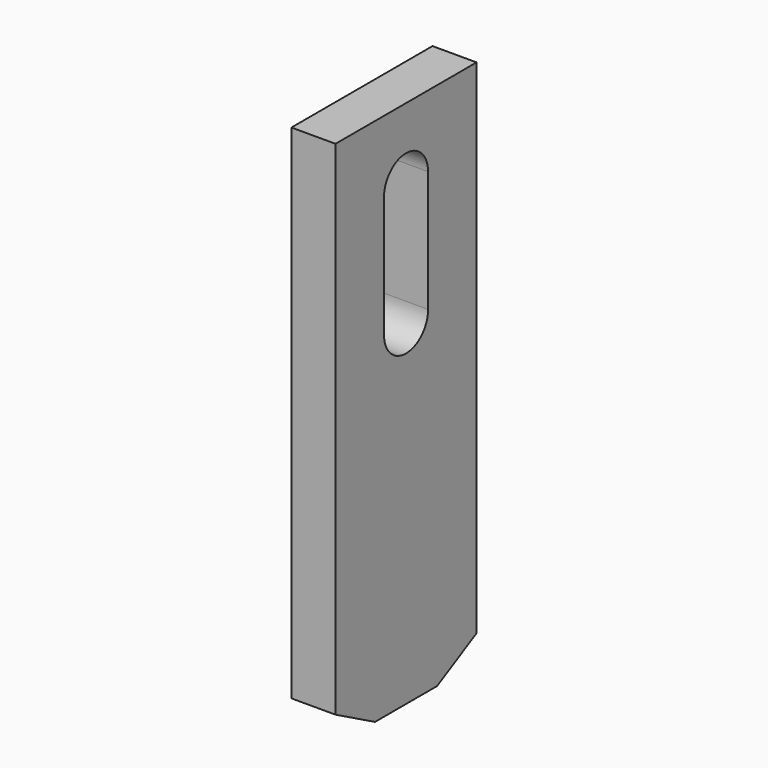
from build123d import *

# Parameters (mm, degrees)
F1_DEPTH = 6.35
F2_SIZE2 = 3.81
F2_SIZE  = 7.112


with BuildPart() as f1:
    # F0 (on Right) → F1 (new body)
    with BuildSketch(Plane.YZ):
        Polygon((26.7912242562, 26.1120563269), (1.3912242562, 26.1120563269), (1.3912242562, -50.0879436731), (26.7912242562, -50.0879436731), (26.7912242562, 3.7854563269), (26.7912242562, 9.8814563269), align=None)
        with BuildLine():
            ThreePointArc((10.1224742562, 15.7933063269), (14.0912242562, 19.7620563269), (18.0599742562, 15.7933063269))
            Line((18.0599742562, 15.7933063269), (18.0599742562, -1.6691936731))
            ThreePointArc((18.0599742562, -1.6691936731), (14.0912242562, -5.6379436731), (10.1224742562, -1.6691936731))
            Line((10.1224742562, -1.6691936731), (10.1224742562, 15.7933063269))
        make_face(mode=Mode.SUBTRACT)
    extrude(amount=F1_DEPTH)

    # F2
    f2_edges = [f1.edges().sort_by_distance(p)[0] for p in [
        (3.175, 1.391224, -50.087944),
        (3.175, 26.791224, -50.087944),
    ]]
    f2_side = f1.faces().sort_by_distance((3.175, 14.091224, -50.087944))[0]
    chamfer(f2_edges, length=F2_SIZE, length2=F2_SIZE2, reference=f2_side)


solid = f1.part
